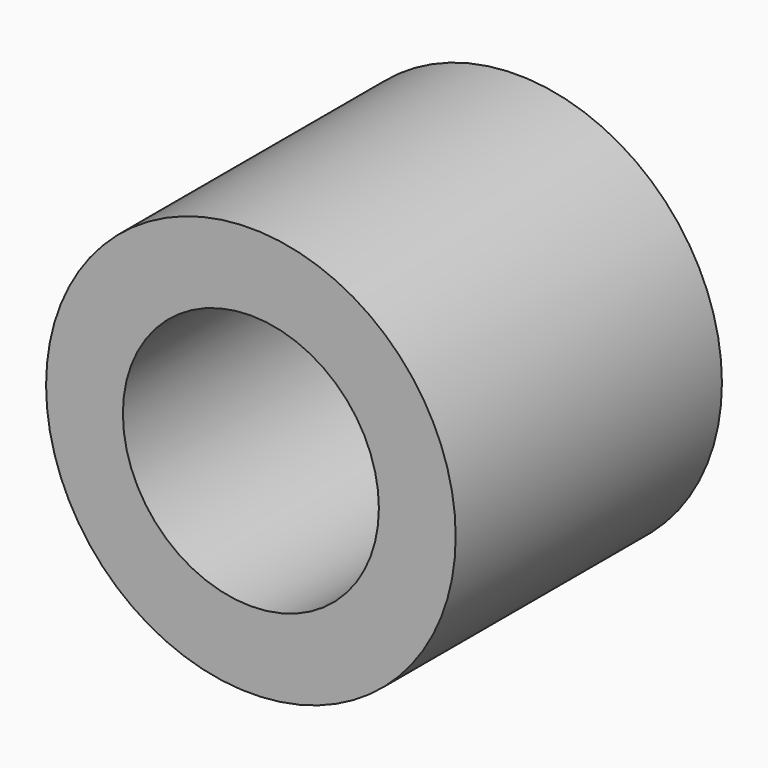
from build123d import *

# Parameters (mm, degrees)
F0_R     = 12.7
F1_DEPTH = 20.6375
F2_R     = 7.9375
F3_DEPTH = 20.6375


# Not quite as in the source:
# - a length typed as a fraction of an inch, garbled in the dataset ("3 / 203.2 mm" for 3/8 in), is restored


with BuildPart() as f1:
    # F0 (on Front) → F1 (new body)
    with BuildSketch(Plane.XZ):
        Circle(F0_R)
    extrude(amount=F1_DEPTH)

    # F2 (on Front) → F3 (cut)
    with BuildSketch(Plane.XZ):
        Circle(F2_R)
    extrude(amount=F3_DEPTH, mode=Mode.SUBTRACT)


solid = f1.part
